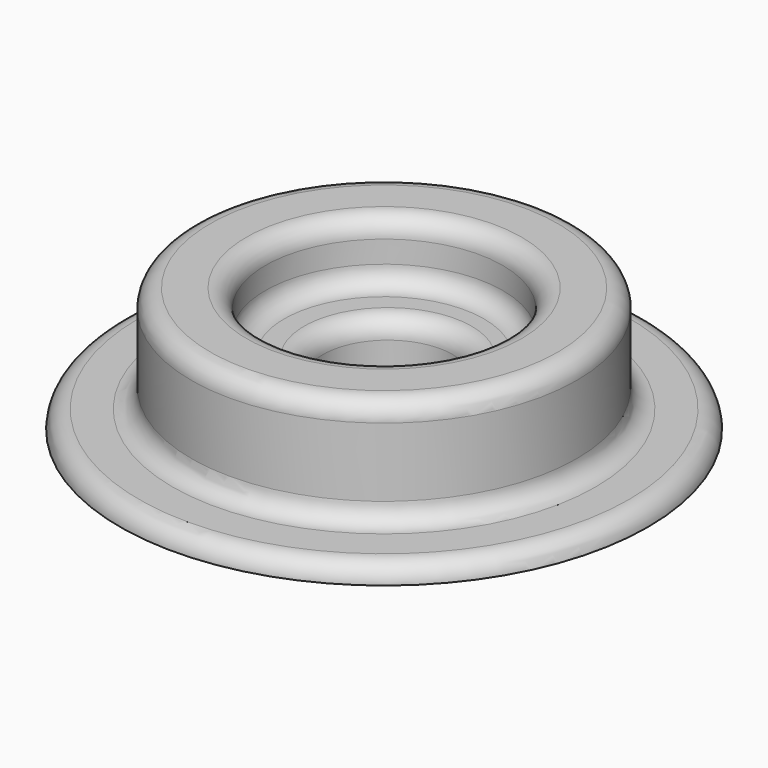
from build123d import *

# Parameters (mm, degrees)
F1_R     = 74.1708430985
F1_R_2   = 45.6987407436
F2_DEPTH = 48
F0_R     = 50
F0_R_2   = 25
F3_DEPTH = 25
F4_R     = 7.2426406871
F1_R_3   = 101.591361741
F5_DEPTH = 7


# Not quite as in the source:
# - a fillet or chamfer that OpenCascade refuses, or shapes differently, is made with other operations: its cross-section is extruded or revolved along the edge and cut away or added


with BuildPart() as f2:
    # F1 (on Top) → F2 (new body)
    with BuildSketch(Plane.XY):
        Circle(F1_R)
        Circle(F1_R_2, mode=Mode.SUBTRACT)
    extrude(amount=F2_DEPTH)

    # F0 (on Top) → F3 (join)
    with BuildSketch(Plane.XY):
        with Locations((1.4469225327, 0)):
            Circle(F0_R)
        with Locations((1.4469225327, 0)):
            Circle(F0_R_2, mode=Mode.SUBTRACT)
    extrude(amount=F3_DEPTH)

    # F4
    f4_edges = [f2.edges().sort_by_distance(p)[0] for p in [
        (-45.698741, 0, 25),
        (-23.553077, 0, 25),
        (-74.170843, 0, 48),
        (-45.698741, 0, 48),
    ]]
    fillet(f4_edges, radius=F4_R)

    # F1 (on Top) → F5 (join)
    with BuildSketch(Plane.XY):
        Circle(F1_R_3)
        Circle(F1_R, mode=Mode.SUBTRACT)
    extrude(amount=F5_DEPTH)

    # F6: fillet of radius 7.2426406871 on 2 edges, made by hand

    # F6_s1 → F6_t2 (revolve)
    with BuildSketch(Plane.XZ):
        with BuildLine():
            ThreePointArc((74.1708430985, 14.2426406871), (76.2921634421, 9.1213203436), (81.4134837857, 7))
            Line((81.4134837857, 7), (74.1708430985, 7))
            Line((74.1708430985, 7), (74.1708430985, 14.2426406871))
        make_face()
    revolve(axis=Axis((0, 0, 7), (0, 0, 1)))

    # F6_s3 → F6_t4 (revolve, cut)
    with BuildSketch(Plane.XZ):
        with BuildLine():
            ThreePointArc((94.3527866313, 7), (99.3875897461, 4.9637593857), (101.591361741, 0))
            Line((101.591361741, 0), (101.591361741, 7))
            Line((101.591361741, 7), (94.3527866313, 7))
        make_face()
    revolve(axis=Axis((0, 0, 7), (0, 0, 1)), mode=Mode.SUBTRACT)


solid = f2.part
